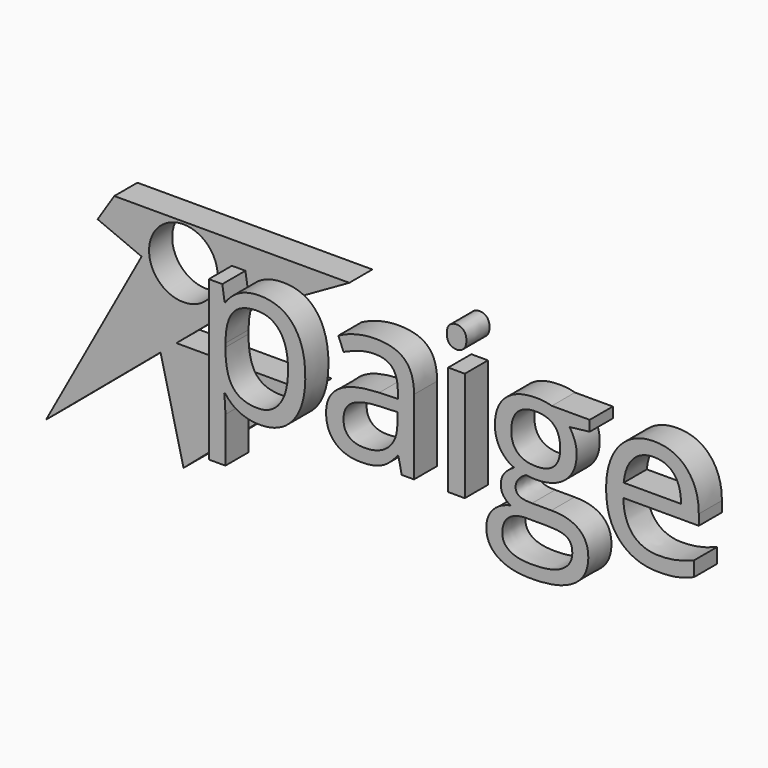
from build123d import *

# Parameters (mm, degrees)
F2_DEPTH     = 25.4
F3_R         = 30.1353781358
F4_DEPTH     = 25.4
F5_TEXT_SIZE = 179.9676981237
F6_DEPTH     = 25.4


# Not quite as in the source:
# - Text() gives the source's letters only with a copy of the font that has no kerning and outlines rounded to 1/6400 em; it was checked with that copy


with BuildPart() as f2:
    # F1 (on Front) → F2 (new body)
    with BuildSketch(Plane.XZ):
        Polygon((2.8730910226, -11.7382635953), (23.1293588877, -94.4970101118), (132.825538516, 0), (16.8044590106, 0), align=None)
        Polygon((-97.6718962193, -96.4552536607), (2.8730910226, -11.7382635953), (0, 0), (-13.7199352813, 57.0234765978), align=None)
        Polygon((0, 0), (2.8730910226, -11.7382635953), (16.8044590106, 0), align=None)
        Polygon((-13.7199352813, 57.0234765978), (0, 0), (51.782527114, 29.4717492071), align=None)
        Polygon((51.782527114, 29.4717492071), (0, 0), (16.8044590106, 0), align=None)
        Polygon((-13.7199352813, 57.0234765978), (51.782527114, 29.4717492071), (168.7524467707, 96.0445553064), (-37.7278625965, 96.0445553064), (-52.3873195052, 73.2877999544), align=None)
    extrude(amount=F2_DEPTH)

    # F3 (on face) → F4 (cut)
    with BuildSketch(Plane.XZ.offset(25.4)):
        with Locations((22.953376174, 63.8025254011)):
            Circle(F3_R)
    extrude(amount=-F4_DEPTH, mode=Mode.SUBTRACT)


with BuildPart() as f6:
    # F5 (on face) → F6 (new body)
    with BuildSketch(Plane.XZ.offset(25.4)):
        with Locations((50.1445308328, -20.6293910742)):
            Text('paige', F5_TEXT_SIZE, font='Open Sans', text_align=(TextAlign.LEFT, TextAlign.BOTTOM))
    extrude(amount=F6_DEPTH)


solid = Compound([f2.part, f6.part])
